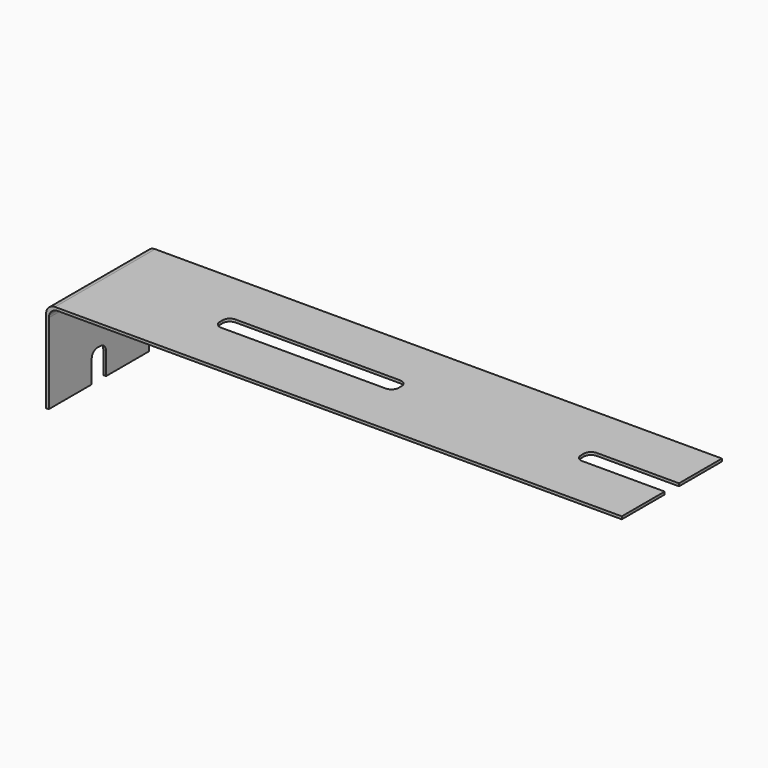
from build123d import *

# Parameters (mm, degrees)
F1_DEPTH = 0.15
F2_DEPTH = 1.9
F3_W     = 0.15
F3_H     = 7
F4_DEPTH = 5
F6_DEPTH = 25
F7_R     = 0.5


# Not quite as in the source:
# - a feature names something its author has since deleted; it is built from what else it names


with BuildPart() as f1:
    # F0 (on Top) → F1 (new body)
    with BuildSketch(Plane.XY):
        with BuildLine():
            Line((10.1, -0.5), (10.1, -3.5))
            Line((10.1, -3.5), (20.2, -3.5))
            Line((20.2, -3.5), (30.3, -3.5))
            Line((30.3, -3.5), (30.3, -0.5))
            Line((30.3, -0.5), (25.7, -0.5))
            ThreePointArc((25.7, -0.5), (25.4171572875, -0.3828427125), (25.3, -0.1))
            Line((25.3, -0.1), (25.3, 0.1))
            ThreePointArc((25.3, 0.1), (25.4171572875, 0.3828427125), (25.7, 0.5))
            Line((25.7, 0.5), (30.3, 0.5))
            Line((30.3, 0.5), (30.3, 3.5))
            Line((30.3, 3.5), (20.2, 3.5))
            Line((20.2, 3.5), (10.1, 3.5))
            Line((10.1, 3.5), (10.1, 0.5))
            Line((10.1, 0.5), (14.7, 0.5))
            ThreePointArc((14.7, 0.5), (14.9828427125, 0.3828427125), (15.1, 0.1))
            Line((15.1, 0.1), (15.1, -0.1))
            ThreePointArc((15.1, -0.1), (14.9828427125, -0.3828427125), (14.7, -0.5))
            Line((14.7, -0.5), (10.1, -0.5))
        make_face()
        with BuildLine():
            Line((0, 3.5), (0, -3.5))
            Line((0, -3.5), (10.1, -3.5))
            Line((10.1, -3.5), (10.1, -0.5))
            Line((10.1, -0.5), (5.5, -0.5))
            ThreePointArc((5.5, -0.5), (5.2171572875, -0.3828427125), (5.1, -0.1))
            Line((5.1, -0.1), (5.1, 0.1))
            ThreePointArc((5.1, 0.1), (5.2171572875, 0.3828427125), (5.5, 0.5))
            Line((5.5, 0.5), (10.1, 0.5))
            Line((10.1, 0.5), (10.1, 3.5))
            Line((10.1, 3.5), (0, 3.5))
        make_face()
    extrude(amount=F1_DEPTH)

    # F2 (add): a face of the model
    f2_faces = [f1.faces().sort_by_distance(p)[0] for p in [
        (0, 0, 0.075),
    ]]
    extrude(f2_faces, amount=F2_DEPTH)

    # F3 (on face) → F4 (join)
    with BuildSketch(Plane(origin=(0, 0, 0), x_dir=(1, 0, 0), z_dir=(0, 0, -1))):
        with Locations((-1.825, 0)):
            Rectangle(F3_W, F3_H)
    extrude(amount=F4_DEPTH)

    # F5 (on face) → F6 (cut)
    with BuildSketch(Plane(origin=(-1.9, 0, 0), x_dir=(0, -1, 0), z_dir=(-1, 0, 0))):
        with BuildLine():
            ThreePointArc((0.5, -3.75), (0.3828427125, -3.4671572875), (0.1, -3.35))
            Line((0.1, -3.35), (-0.1, -3.35))
            ThreePointArc((-0.1, -3.35), (-0.3828427125, -3.4671572875), (-0.5, -3.75))
            Line((-0.5, -3.75), (-0.5, -5))
            Line((-0.5, -5), (0.5, -5))
            Line((0.5, -5), (0.5, -3.75))
        make_face()
    extrude(amount=-F6_DEPTH, mode=Mode.SUBTRACT)

    # F7
    f7_edges = [f1.edges().sort_by_distance(p)[0] for p in [
        (-1.9, 0, 0.15),
        (-1.75, 0, 0),
    ]]
    fillet(f7_edges, radius=F7_R)


solid = f1.part
